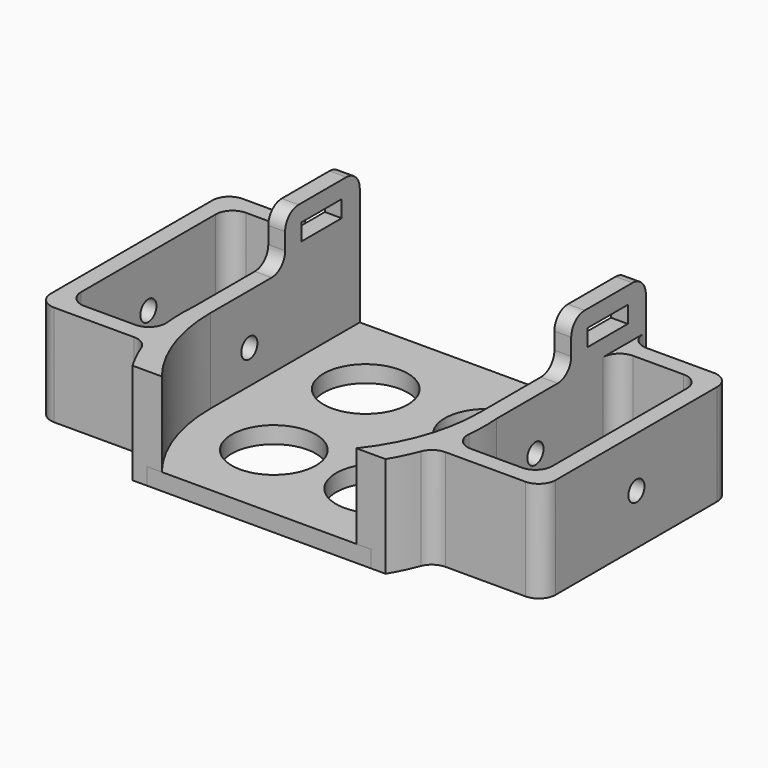
from build123d import *

# Parameters (mm, degrees)
F1_DEPTH  = 30
F3_DEPTH  = 5
F4_R      = 3
F5_DEPTH  = 35
F6_R      = 3
F7_DEPTH  = 35
F9_W      = 27.7209319142
F9_H      = 15
F9_W_2    = 15
F9_H_2    = 5
F10_DEPTH = 5
F11_R     = 5
F12_R     = 5
F13_R     = 5
F13_2_R   = 5
F14_R     = 5
F15_W     = 27.7209319142
F15_H     = 15
F15_W_2   = 15
F15_H_2   = 5
F16_DEPTH = 5
F17_R     = 5
F18_R     = 12.5
F19_DEPTH = 5


with BuildPart() as f1:
    # F0 (on Top) → F1 (new body)
    with BuildSketch(Plane.XY):
        with BuildLine():
            Line((-45, 44.4425949542), (-45, 0))
            ThreePointArc((-45, 0), (-45.066266446, -7.8147796829), (-44.0046991035, -15.5574050458))
            ThreePointArc((-44.0046991035, -15.5574050458), (-43.4089049923, -18.0730910814), (-42.6934813561, -20.5574050458))
            ThreePointArc((-42.6934813561, -20.5574050458), (-40.475443237, -26.4101305765), (-37.5955815851, -31.9671519101))
            Line((-37.5955815851, -31.9671519101), (-28.8889932035, -31.9671519101))
            ThreePointArc((-28.8889932035, -31.9671519101), (-37.1430686541, -16.9215341597), (-40, 0))
            Line((-40, 0), (-40, 55.4418638284))
            Line((-40, 55.4418638284), (-45, 55.4418638284))
            Line((-45, 55.4418638284), (-45, 49.4425949542))
            Line((-45, 49.4425949542), (-45, 44.4425949542))
        make_face()
        with BuildLine():
            ThreePointArc((-42.6934813561, -20.5574050458), (-43.4089049923, -18.0730910814), (-44.0046991035, -15.5574050458))
            Line((-44.0046991035, -15.5574050458), (-70, -15.5574050458))
            Line((-70, -15.5574050458), (-70, 44.4425949542))
            Line((-70, 44.4425949542), (-45, 44.4425949542))
            Line((-45, 44.4425949542), (-45, 49.4425949542))
            Line((-45, 49.4425949542), (-75, 49.4425949542))
            Line((-75, 49.4425949542), (-75, -20.5574050458))
            Line((-75, -20.5574050458), (-42.6934813561, -20.5574050458))
        make_face()
    extrude(amount=F1_DEPTH)

    # F6 (on face) → F7 (cut)
    with BuildSketch(Plane(origin=(-75, 0, 0), x_dir=(0, -1, 0), z_dir=(-1, 0, 0))):
        with Locations((-14.4425949542, 15)):
            Circle(F6_R)
    extrude(amount=-F7_DEPTH, mode=Mode.SUBTRACT)

    # F9 (on face) → F10 (join)
    with BuildSketch(Plane(origin=(-45, 0, 0), x_dir=(0, -1, 0), z_dir=(-1, 0, 0))):
        with Locations((-41.5813978713, 37.5)):
            Rectangle(F9_W, F9_H)
        with Locations((-41.235268414, 37.4656194448)):
            Rectangle(F9_W_2, F9_H_2, mode=Mode.SUBTRACT)
    extrude(amount=-F10_DEPTH)

    # F11
    f11_edges = [f1.edges().sort_by_distance(p)[0] for p in [
        (-75, 49.442595, 15),
        (-75, -20.557405, 15),
    ]]
    fillet(f11_edges, radius=F11_R)

    # F13
    f13_edges = [f1.edges().sort_by_distance(p)[0] for p in [
        (-70, 44.442595, 15),
        (-70, -15.557405, 15),
        (-45, 44.442595, 15),
        (-44.004699, -15.557405, 15),
        (-42.693481, -20.557405, 15),
        (-45, 49.442595, 15),
        (-42.5, 27.720932, 30),
    ]]
    fillet(f13_edges, radius=F13_R)

    # F14
    f14_edges = [f1.edges().sort_by_distance(p)[0] for p in [
        (-42.5, 55.441864, 45),
        (-42.5, 27.720932, 45),
    ]]
    fillet(f14_edges, radius=F14_R)


with BuildPart() as f1b:
    # F0 (on Top) → F1, piece 2 (new body)
    with BuildSketch(Plane.XY):
        with BuildLine():
            ThreePointArc((44.0046991035, -15.5574050458), (45.066266446, -7.8147796829), (45, 0))
            Line((45, 0), (45, 44.4425949542))
            Line((45, 44.4425949542), (45, 49.4425949542))
            Line((45, 49.4425949542), (45, 55.4418638284))
            Line((45, 55.4418638284), (40, 55.4418638284))
            Line((40, 55.4418638284), (40, 0))
            ThreePointArc((40, 0), (37.1430686541, -16.9215341597), (28.8889932035, -31.9671519101))
            Line((28.8889932035, -31.9671519101), (37.5955815851, -31.9671519101))
            ThreePointArc((37.5955815851, -31.9671519101), (40.475443237, -26.4101305765), (42.6934813561, -20.5574050458))
            ThreePointArc((42.6934813561, -20.5574050458), (43.4089049923, -18.0730910814), (44.0046991035, -15.5574050458))
        make_face()
        with BuildLine():
            Line((45, 49.4425949542), (45, 44.4425949542))
            Line((45, 44.4425949542), (70, 44.4425949542))
            Line((70, 44.4425949542), (70, -15.5574050458))
            Line((70, -15.5574050458), (44.0046991035, -15.5574050458))
            ThreePointArc((44.0046991035, -15.5574050458), (43.4089049923, -18.0730910814), (42.6934813561, -20.5574050458))
            Line((42.6934813561, -20.5574050458), (75, -20.5574050458))
            Line((75, -20.5574050458), (75, 49.4425949542))
            Line((75, 49.4425949542), (45, 49.4425949542))
        make_face()
    extrude(amount=F1_DEPTH)

    # F4 (on face) → F5 (cut)
    with BuildSketch(Plane.YZ.offset(75)):
        with Locations((14.4425949542, 15)):
            Circle(F4_R)
    extrude(amount=-F5_DEPTH, mode=Mode.SUBTRACT)

    # F12
    f12_edges = [f1b.edges().sort_by_distance(p)[0] for p in [
        (75, -20.557405, 15),
        (75, 49.442595, 15),
    ]]
    fillet(f12_edges, radius=F12_R)

    # F13#2
    f13_2_edges = [f1b.edges().sort_by_distance(p)[0] for p in [
        (70, 44.442595, 15),
        (70, -15.557405, 15),
        (45, 44.442595, 15),
        (44.004699, -15.557405, 15),
        (42.693481, -20.557405, 15),
        (45, 49.442595, 15),
    ]]
    fillet(f13_2_edges, radius=F13_2_R)

    # F15 (on face) → F16 (join)
    with BuildSketch(Plane.YZ.offset(45)):
        with Locations((41.5813978713, 37.5)):
            Rectangle(F15_W, F15_H)
        with Locations((41.235268414, 37.4656194448)):
            Rectangle(F15_W_2, F15_H_2, mode=Mode.SUBTRACT)
    extrude(amount=-F16_DEPTH)

    # F17
    f17_edges = [f1b.edges().sort_by_distance(p)[0] for p in [
        (42.5, 55.441864, 45),
        (42.5, 27.720932, 45),
        (42.5, 27.720932, 30),
    ]]
    fillet(f17_edges, radius=F17_R)


with BuildPart() as f3:
    # F2 (on face) → F3 (new body)
    with BuildSketch(Plane(origin=(0, 0, 0), x_dir=(1, 0, 0), z_dir=(0, 0, -1))):
        Polygon((-42.5, 0), (-42.5, -55.4418638284), (0, -55.4418638284), (0, 31.9671519101), (-33.2422873943, 31.9671519101), align=None)
        Polygon((0, 31.9671519101), (0, -55.4418638284), (42.5, -55.4418638284), (42.5, 0), (33.2422873943, 31.9671519101), align=None)
    extrude(amount=-F3_DEPTH)

    # F18 (on face) → F19 (cut)
    with BuildSketch(Plane.XY.offset(5)):
        with Locations((-17.9911866391, 30.1519593033)):
            Circle(F18_R)
        with Locations((-15.5046174286, -7.0962243824)):
            Circle(F18_R)
        with Locations((17.9911866391, 30.1519593033)):
            Circle(F18_R)
        with Locations((15.5046174286, -7.0962243824)):
            Circle(F18_R)
    extrude(amount=-F19_DEPTH, mode=Mode.SUBTRACT)


solid = Compound([f1.part, f1b.part, f3.part])
